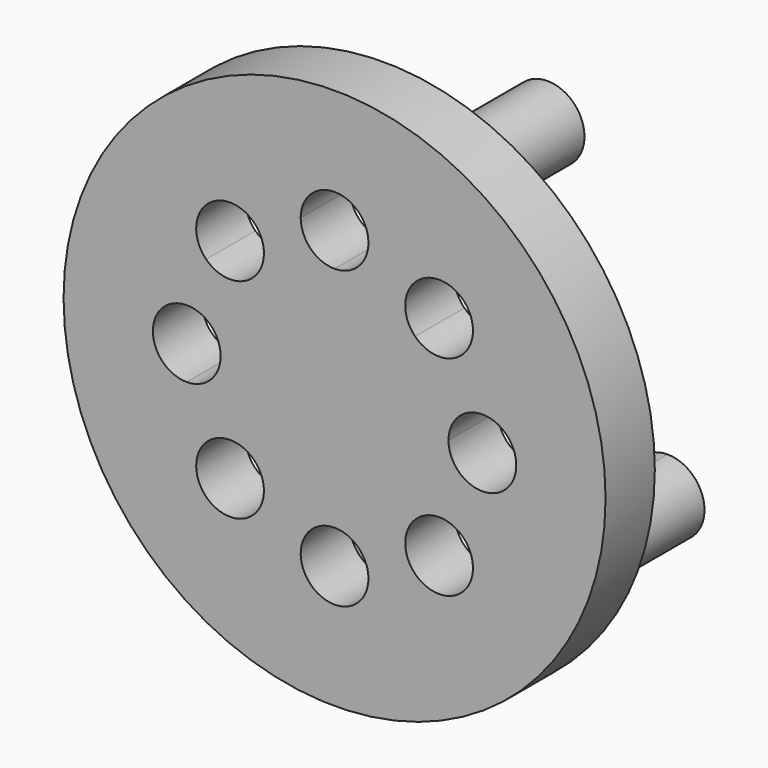
from build123d import *

# Parameters (mm, degrees)
F0_R            = 22
F1_DEPTH        = 5
F3_DEPTH        = 25
F3_COPIES_COUNT = 8
F5_DEPTH        = 8
F5_COPIES_COUNT = 4


# Not quite as in the source:
# - a pattern or mirror of a feature is missing from the dataset's text; its kind, count and spacing are read off the source's solid
# - a feature names something its author has since deleted; it is built from what else it names


with BuildPart() as f1:
    # F0 (on Front) → F1 (new body)
    with BuildSketch(Plane.XZ):
        Circle(F0_R)
    extrude(amount=F1_DEPTH)

    # F2 (on face) → F3 (cut)
    with BuildSketch(Plane.XZ.offset(5)):
        with BuildLine():
            ThreePointArc((0, -9.25), (-1.9445436483, -13.9445436483), (2.75, -12))
            ThreePointArc((2.75, -12), (1.9445436483, -10.0554563517), (0, -9.25))
        make_face()
    f3 = extrude(amount=-F3_DEPTH, mode=Mode.SUBTRACT)

    # F3_copies: F3 ×8 about axis
    f3_copies_axis = Axis((0, 0, 0), (0, 1, 0))
    for i in range(1, F3_COPIES_COUNT):
        add(f3.rotate(f3_copies_axis, i * 360 / F3_COPIES_COUNT), mode=Mode.SUBTRACT)

    # F4 (on face) → F5 (join)
    with BuildSketch(Plane(origin=(0, 0, 0), x_dir=(-1, 0, 0), z_dir=(0, 1, 0))):
        with BuildLine():
            ThreePointArc((-5.7402514855, 13.8581929877), (-4.3938929457, 14.9631208861), (-3.8883017826, 16.6298315852))
            ThreePointArc((-3.8883017826, 16.6298315852), (-9.3827106195, 18.2965422843), (-5.7402514855, 13.8581929877))
        make_face()
    f5 = extrude(amount=F5_DEPTH)

    # F5_copies: F5 ×4 about axis
    f5_copies_axis = Axis((0, 0, 0), (0, 1, 0))
    for i in range(1, F5_COPIES_COUNT):
        add(f5.rotate(f5_copies_axis, i * 360 / F5_COPIES_COUNT))


solid = f1.part
